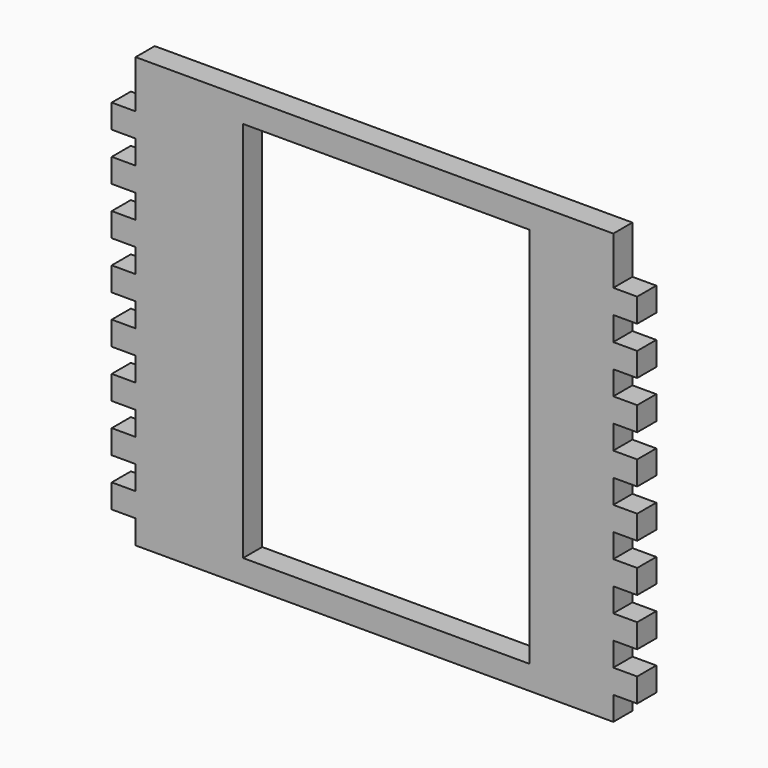
from build123d import *

# Parameters (mm, degrees)
F0_W     = 3.175
F0_H     = 3.175
F1_DEPTH = 3.175


# Not quite as in the source:
# - a feature names something its author has since deleted; it is built from what else it names


with BuildPart() as f1:
    # F0 (on Front) → F1 (new body)
    with BuildSketch(Plane.XZ):
        Polygon((-56.6817452915, 14.4236114298), (-56.6817452915, 11.2486114298), (-53.5067452915, 11.2486114298), (-42.3942452915, 11.2486114298), (-23.3442452915, 11.2486114298), (-4.2942452915, 11.2486114298), (6.8182547085, 11.2486114298), (6.8182547085, 14.4236114298), align=None)
        with Locations((-55.0942452915, 9.6611114298)):
            Rectangle(F0_W, F0_H)
        with Locations((-58.2692452915, 6.4861114298)):
            Rectangle(F0_W, F0_H)
        Polygon((-42.3942452915, 11.2486114298), (-53.5067452915, 11.2486114298), (-53.5067452915, 8.0736114298), (-53.5067452915, 4.8986114298), (-53.5067452915, 1.7236114298), (-53.5067452915, -1.4513885702), (-53.5067452915, -4.6263885702), (-53.5067452915, -7.8013885702), (-53.5067452915, -10.9763885702), (-53.5067452915, -14.1513885702), (-53.5067452915, -17.3263885702), (-53.5067452915, -20.5013885702), (-53.5067452915, -23.6763885702), (-53.5067452915, -26.8513885702), (-53.5067452915, -30.0263885702), (-53.5067452915, -33.2013885702), (-53.5067452915, -36.3763885702), (-53.5067452915, -39.5513885702), (-42.3942452915, -39.5513885702), align=None)
        with Locations((-55.0942452915, 6.4861114298)):
            Rectangle(F0_W, F0_H)
        with Locations((-55.0942452915, 3.3111114298)):
            Rectangle(F0_W, F0_H)
        with Locations((-58.2692452915, 0.1361114298)):
            Rectangle(F0_W, F0_H)
        Polygon((-23.3442452915, -39.5513885702), (-42.3942452915, -39.5513885702), (-53.5067452915, -39.5513885702), (-53.5067452915, -42.7263885702), (6.8182547085, -42.7263885702), (6.8182547085, -39.5513885702), (-4.2942452915, -39.5513885702), align=None)
        Polygon((6.8182547085, 8.0736114298), (6.8182547085, 11.2486114298), (-4.2942452915, 11.2486114298), (-4.2942452915, -39.5513885702), (6.8182547085, -39.5513885702), (6.8182547085, -36.3763885702), (6.8182547085, -33.2013885702), (6.8182547085, -30.0263885702), (6.8182547085, -26.8513885702), (6.8182547085, -23.6763885702), (6.8182547085, -20.5013885702), (6.8182547085, -17.3263885702), (6.8182547085, -14.1513885702), (6.8182547085, -10.9763885702), (6.8182547085, -7.8013885702), (6.8182547085, -4.6263885702), (6.8182547085, -1.4513885702), (6.8182547085, 1.7236114298), (6.8182547085, 4.8986114298), align=None)
        with Locations((-55.0942452915, 0.1361114298)):
            Rectangle(F0_W, F0_H)
        with Locations((-55.0942452915, -41.1388885702)):
            Rectangle(F0_W, F0_H)
        with Locations((-55.0942452915, -37.9638885702)):
            Rectangle(F0_W, F0_H)
        with Locations((8.4057547085, 6.4861114298)):
            Rectangle(F0_W, F0_H)
        with Locations((-55.0942452915, -3.0388885702)):
            Rectangle(F0_W, F0_H)
        with Locations((-58.2692452915, -6.2138885702)):
            Rectangle(F0_W, F0_H)
        with Locations((-58.2692452915, -37.9638885702)):
            Rectangle(F0_W, F0_H)
        with Locations((-55.0942452915, -34.7888885702)):
            Rectangle(F0_W, F0_H)
        with Locations((-55.0942452915, -6.2138885702)):
            Rectangle(F0_W, F0_H)
        with Locations((8.4057547085, -37.9638885702)):
            Rectangle(F0_W, F0_H)
        with Locations((-55.0942452915, -31.6138885702)):
            Rectangle(F0_W, F0_H)
        with Locations((8.4057547085, 0.1361114298)):
            Rectangle(F0_W, F0_H)
        with Locations((-55.0942452915, -9.3888885702)):
            Rectangle(F0_W, F0_H)
        with Locations((-58.2692452915, -12.5638885702)):
            Rectangle(F0_W, F0_H)
        with Locations((-58.2692452915, -31.6138885702)):
            Rectangle(F0_W, F0_H)
        with Locations((-55.0942452915, -28.4388885702)):
            Rectangle(F0_W, F0_H)
        with Locations((-55.0942452915, -12.5638885702)):
            Rectangle(F0_W, F0_H)
        with Locations((8.4057547085, -31.6138885702)):
            Rectangle(F0_W, F0_H)
        with Locations((-55.0942452915, -25.2638885702)):
            Rectangle(F0_W, F0_H)
        with Locations((8.4057547085, -6.2138885702)):
            Rectangle(F0_W, F0_H)
        with Locations((-55.0942452915, -15.7388885702)):
            Rectangle(F0_W, F0_H)
        with Locations((-58.2692452915, -18.9138885702)):
            Rectangle(F0_W, F0_H)
        with Locations((-58.2692452915, -25.2638885702)):
            Rectangle(F0_W, F0_H)
        with Locations((-55.0942452915, -22.0888885702)):
            Rectangle(F0_W, F0_H)
        with Locations((-55.0942452915, -18.9138885702)):
            Rectangle(F0_W, F0_H)
        with Locations((8.4057547085, -25.2638885702)):
            Rectangle(F0_W, F0_H)
        with Locations((8.4057547085, -12.5638885702)):
            Rectangle(F0_W, F0_H)
        with Locations((8.4057547085, -18.9138885702)):
            Rectangle(F0_W, F0_H)
    extrude(amount=F1_DEPTH)


solid = f1.part
